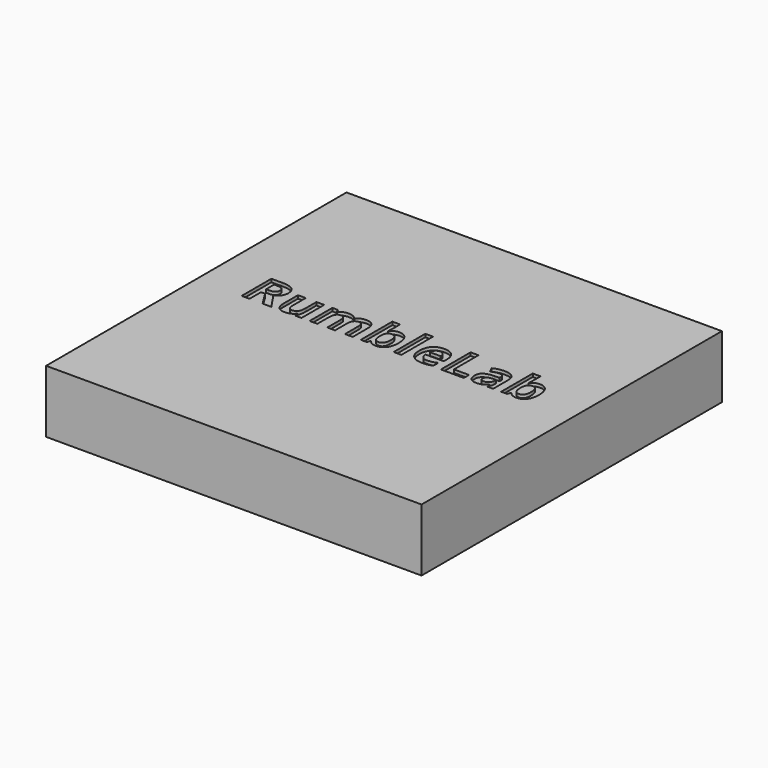
from build123d import *

# Parameters (mm, degrees)
F0_W         = 304.8
F0_H         = 304.8
F1_DEPTH     = 50.8
F2_TEXT_SIZE = 42.24999963
F3_DEPTH     = 2.54


# Not quite as in the source:
# - Text() gives the source's letters only with a copy of the font that has no kerning and outlines rounded to 1/6400 em; it was checked with that copy


with BuildPart() as f1:
    # F0 (on Top) → F1 (new body)
    with BuildSketch(Plane.XY):
        Rectangle(F0_W, F0_H)
    extrude(amount=F1_DEPTH)

    # F2 (on face) → F3 (cut)
    with BuildSketch(Plane.XY.offset(50.8)):
        with Locations((-119.3529481734, 0)):
            Text('RumbleLab', F2_TEXT_SIZE, font='Open Sans', font_style=FontStyle.BOLD, text_align=(TextAlign.LEFT, TextAlign.BOTTOM))
    extrude(amount=-F3_DEPTH, mode=Mode.SUBTRACT)


solid = f1.part
